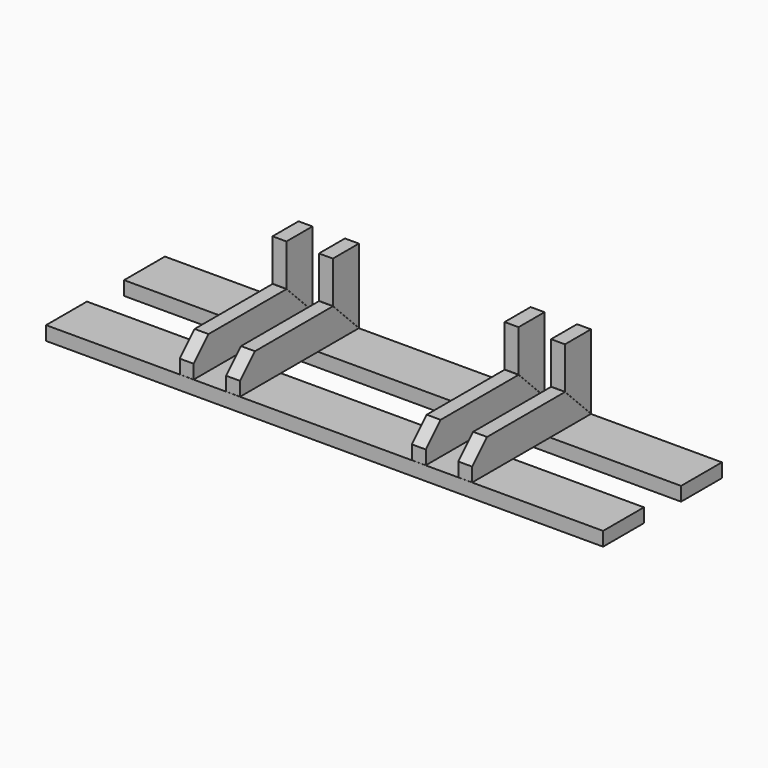
from build123d import *

# Parameters (mm, degrees)
F0_W      = 1524
F0_H      = 139.7
F1_DEPTH  = 38.1
F6_W      = 406.4
F6_H      = 88.9
F7_DEPTH  = 38.1
F9_SIZE   = 50.8
F10_SIZE  = 88.89999
F13_W     = 88.9
F13_H     = 203.2
F14_DEPTH = 38.1
F15_SIZE  = 88.89999


# Not quite as in the source:
# - a fillet or chamfer is up to 0.001 mm smaller than in the source, because OpenCascade refuses the exact size


with BuildPart() as f1:
    # F0 (on Top) → F1 (new body)
    with BuildSketch(Plane.XY):
        with Locations((15.5021820764, 32.6323900372)):
            Rectangle(F0_W, F0_H)
    extrude(amount=F1_DEPTH)


with BuildPart() as f2_1:
    # F2: copy of F1
    add(f1.part)


with BuildPart() as f2_1_1:
    # F3: moved
    add(f2_1.part.moved(Location((0, 203.2, 0))))


with BuildPart() as f1_1:
    # F4: moved
    add(f1.part.moved(Location((0, -152.4, 0))))


with BuildPart() as f2_1_2:
    # F5: moved
    add(f2_1_1.part.moved(Location((0, -114.3, 0))))


with BuildPart() as f7:
    # F6 (on Right) → F7 (new body)
    with BuildSketch(Plane.YZ):
        with Locations((10.0957566703, 44.45)):
            Rectangle(F6_W, F6_H)
    extrude(amount=F7_DEPTH)


with BuildPart() as f7_1:
    # F8: moved
    add(f7.part.moved(Location((0, 0, 38.1))))

    # F9
    f9_edges = [f7_1.edges().sort_by_distance(p)[0] for p in [
        (19.05, -193.104243, 127),
    ]]
    chamfer(f9_edges, length=F9_SIZE)

    # F10 (size 88.9 in the source; OpenCascade refuses exactly that, so slightly less here)
    f10_edges = [f7_1.edges().sort_by_distance(p)[0] for p in [
        (19.05, 213.295757, 127),
    ]]
    chamfer(f10_edges, length=F10_SIZE)


with BuildPart() as f2_1_3:
    # F11: moved
    add(f2_1_2.part.moved(Location((0, 21.59, 0))))


with BuildPart() as f1_2:
    # F12: moved
    add(f1_1.part.moved(Location((0, -3.81, 0))))


with BuildPart() as f14:
    # F13 (on Right) → F14 (new body)
    with BuildSketch(Plane.YZ):
        with Locations((204.4389173388, -3.0202485595)):
            Rectangle(F13_W, F13_H)
    extrude(amount=F14_DEPTH)

    # F15 (size 88.9 in the source; OpenCascade refuses exactly that, so slightly less here)
    f15_edges = [f14.edges().sort_by_distance(p)[0] for p in [
        (19.05, 159.988917, -104.620249),
    ]]
    chamfer(f15_edges, length=F15_SIZE)


with BuildPart() as f14_1:
    # F16: moved
    add(f14.part.moved(Location((0, -35.814, 143.256))))


with BuildPart() as f17_1:
    # F17: copy of F7
    add(f7_1.part.moved(Location((-381, 0, 0))))


with BuildPart() as f18_1:
    # F18: copy of F14
    add(f14_1.part.moved(Location((-381, 0, 0))))


with BuildPart() as f7_2:
    # F19: moved
    add(f7_1.part.moved(Location((-254, 0, 0))))


with BuildPart() as f14_2:
    # F20: moved
    add(f14_1.part.moved(Location((-254, 0, 0))))


with BuildPart() as f21_1:
    # F21: copy of F17_1
    add(f17_1.part.moved(Location((635, 0, 0))))


with BuildPart() as f22_1:
    # F22: copy of F18_1
    add(f18_1.part.moved(Location((635, 0, 0))))


with BuildPart() as f23_1:
    # F23: copy of F7
    add(f7_2.part.moved(Location((635, 0, 0))))


with BuildPart() as f24_1:
    # F24: copy of F14
    add(f14_2.part.moved(Location((635, 0, 0))))


solid = Compound([f2_1_3.part, f1_2.part, f17_1.part, f18_1.part, f7_2.part, f14_2.part, f21_1.part, f22_1.part, f23_1.part, f24_1.part])
